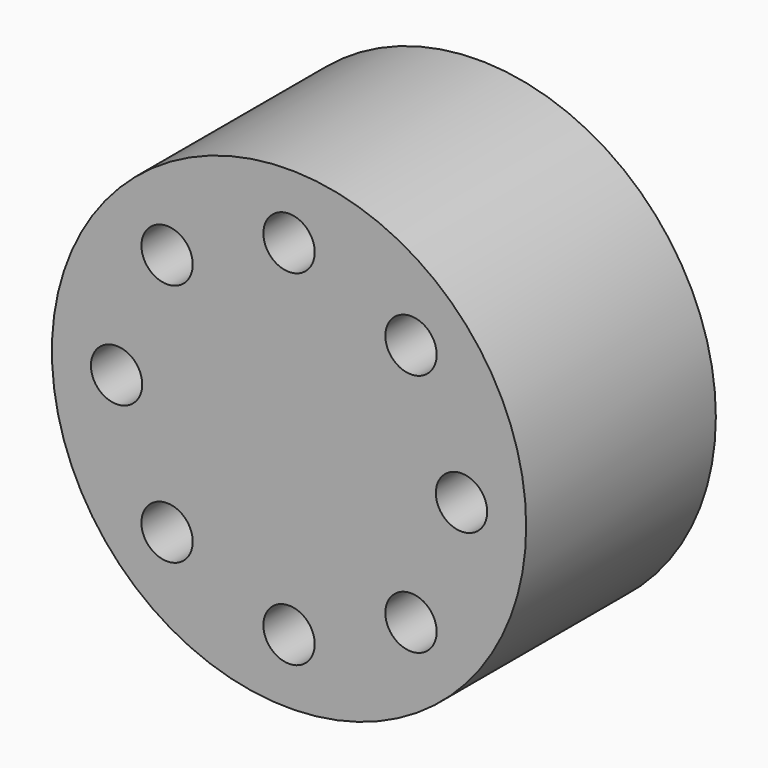
from build123d import *

# Parameters (mm, degrees)
F0_R           = 25.4061794045
F1_DEPTH       = 25.4
F2_D           = 5.5
F2_CBORE_D     = 9.75
F2_CBORE_DEPTH = 5


with BuildPart() as f1:
    # F0 (on Front) → F1 (new body)
    with BuildSketch(Plane.XZ):
        Circle(F0_R)
    extrude(amount=F1_DEPTH)

    # F2 (through all)
    with Locations(Plane(origin=(0, 0, 0), x_dir=(1, 0, 0), z_dir=(0, 1, 0))):
        with Locations((0, -18.4791404754), (-13.0667255406, -13.0667255406), (-18.4791404754, 0), (-13.0667255406, 13.0667255406), (0, 18.4791404754), (13.0667255406, 13.0667255406), (18.4791404754, 0), (13.0667255406, -13.0667255406)):
            CounterBoreHole(F2_D / 2, F2_CBORE_D / 2, F2_CBORE_DEPTH)


solid = f1.part
